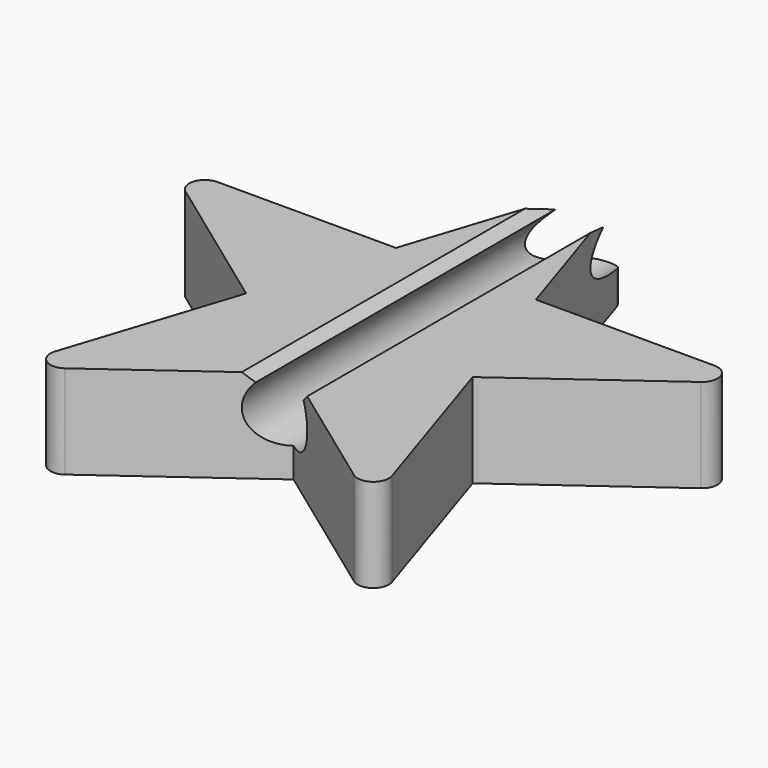
from build123d import *

# Parameters (mm, degrees)
F1_DEPTH      = 3
F2_W          = 4
F2_H          = 6.1803398875
F3_DEPTH      = 1
F5_DEPTH      = 10.001
F5_DEPTH_BACK = 8.0911699437
F6_R          = 0.5
F7_T1_DEPTH   = 13.5993141484
F8_DEPTH      = 1


# Not quite as in the source:
# - a fillet or chamfer that OpenCascade refuses, or shapes differently, is made with other operations: its cross-section is extruded or revolved along the edge and cut away or added


with BuildPart() as f1:
    # F0 (on Top) → F1 (new body)
    with BuildSketch(Plane.XY):
        Polygon((3.63271264, -1.1803398875), (9.510565163, 3.0901699437), (2.2451398829, 3.0901699437), align=None)
        Polygon((3.63271264, -1.1803398875), (2.2451398829, 3.0901699437), (-2.2451398829, 3.0901699437), (-3.63271264, -1.1803398875), (0, -3.8196601125), align=None)
        Polygon((-2.2451398829, 3.0901699437), (2.2451398829, 3.0901699437), (0, 10), align=None)
        Polygon((5.8778525229, -8.0901699437), (3.63271264, -1.1803398875), (0, -3.8196601125), align=None)
        Polygon((-3.63271264, -1.1803398875), (-2.2451398829, 3.0901699437), (-9.510565163, 3.0901699437), align=None)
        Polygon((-5.8778525229, -8.0901699437), (0, -3.8196601125), (-3.63271264, -1.1803398875), align=None)
    extrude(amount=F1_DEPTH)

    # F2 (on face) → F3 (join)
    with BuildSketch(Plane.XY.offset(3)):
        Polygon((3.63271264, -1.1803398875), (9.510565163, 3.0901699437), (2.2451398829, 3.0901699437), (0, 10), (-2.2451398829, 3.0901699437), (-9.510565163, 3.0901699437), (-3.63271264, -1.1803398875), (-5.8778525229, -8.0901699437), (0, -3.8196601125), (5.8778525229, -8.0901699437), align=None)
        Rectangle(F2_W, F2_H, mode=Mode.SUBTRACT)
        Rectangle(F2_W, F2_H)
    extrude(amount=F3_DEPTH)

    # F4 (on Front) → F5 (cut, two sides)
    with BuildSketch(Plane.XZ) as f5_sk:
        with BuildLine():
            ThreePointArc((-0.75, 3.7348469228), (-0.3968626967, 2.0278888952), (1.05, 3))
            ThreePointArc((1.05, 3), (0.9721111048, 3.3968626967), (0.75, 3.7348469228))
            ThreePointArc((0.75, 3.7348469228), (0, 4.05), (-0.75, 3.7348469228))
        make_face()
        with BuildLine():
            ThreePointArc((-0.75, 3.7348469228), (0, 4.05), (0.75, 3.7348469228))
            Line((0.75, 3.7348469228), (0.75, 5))
            Line((0.75, 5), (-0.75, 5))
            Line((-0.75, 5), (-0.75, 3.7348469228))
        make_face()
    extrude(amount=-F5_DEPTH, mode=Mode.SUBTRACT)
    extrude(f5_sk.sketch, amount=F5_DEPTH_BACK, mode=Mode.SUBTRACT)

    # F6
    f6_edges = [f1.edges().sort_by_distance(p)[0] for p in [
        (5.877853, -8.09017, 2),
        (9.510565, 3.09017, 2),
        (0, 10, 0.975),
        (-9.510565, 3.09017, 2),
        (-5.877853, -8.09017, 2),
    ]]
    fillet(f6_edges, radius=F6_R)

    # F7: chamfer of 0.3 on 2 edges, made by hand

    # F7_s2 → F7_t1 (cut)
    with BuildSketch(Plane.XZ.offset(-8.4632422435)):
        Polygon((-0.75, 3.7), (-1.05, 4), (-0.75, 4), align=None)
        Polygon((1.05, 4), (0.75, 3.7), (0.75, 4), align=None)
    extrude(amount=F7_T1_DEPTH, mode=Mode.SUBTRACT)

    # F8 (cut): a face of the model
    f8_faces = [f1.faces().sort_by_distance(p)[0] for p in [
        (0, 0, 0),
    ]]
    extrude(f8_faces, amount=-F8_DEPTH, mode=Mode.SUBTRACT)


solid = f1.part
